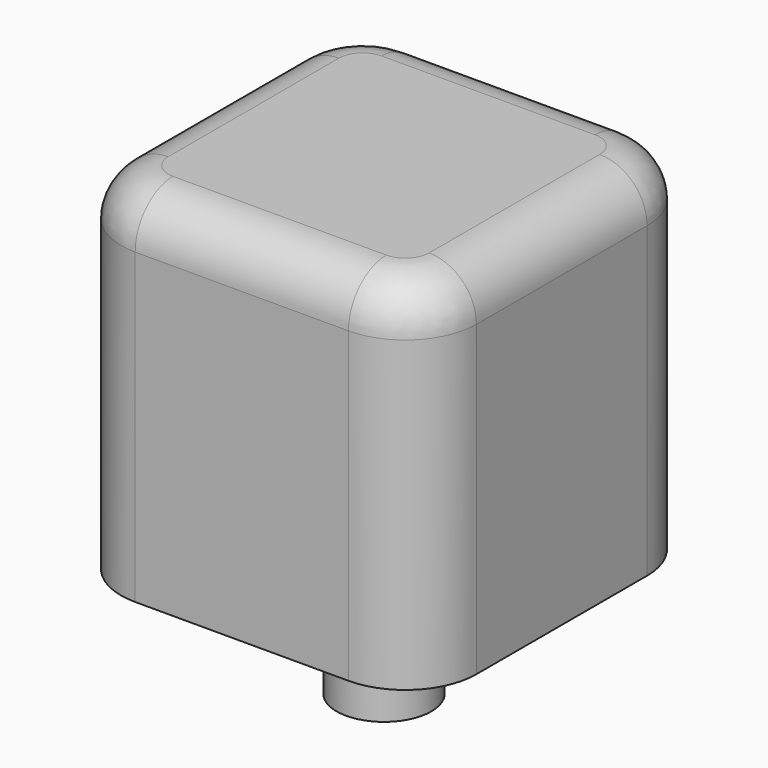
from build123d import *

# Parameters (mm, degrees)
F0_W         = 19.05
F0_H         = 19.05
F1_DEPTH     = 19.05
F2_R         = 2.54
F3_T1_DEPTH  = 28.575
F3_T4_ANGLE  = 90
F3_T6_ANGLE  = 90
F3_T8_ANGLE  = 90
F3_T10_ANGLE = 90
F4_R         = 2.54
F5_DEPTH     = 6.35


# Not quite as in the source:
# - a fillet or chamfer that OpenCascade refuses, or shapes differently, is made with other operations: its cross-section is extruded or revolved along the edge and cut away or added


with BuildPart() as f1:
    # F0 (on Top) → F1 (new body)
    with BuildSketch(Plane.XY):
        with Locations((-40.0474531332, 35.1082887501)):
            Rectangle(F0_W, F0_H)
    extrude(amount=F1_DEPTH)

    # F2
    f2_edges = [f1.edges().sort_by_distance(p)[0] for p in [
        (-40.047453, 44.633289, 19.05),
        (-49.572453, 35.108289, 19.05),
        (-40.047453, 25.583289, 19.05),
        (-30.522453, 35.108289, 19.05),
    ]]
    fillet(f2_edges, radius=F2_R)

    # F3: fillet of radius 3.81 on 4 edges, made by hand

    # F3_s2 → F3_t1 (cut)
    with BuildSketch(Plane.XY.offset(-9.525)):
        with BuildLine():
            ThreePointArc((-49.5724531332, 29.3932887501), (-48.4565299695, 26.6992119137), (-45.7624531332, 25.5832887501))
            Line((-45.7624531332, 25.5832887501), (-49.5724531332, 25.5832887501))
            Line((-49.5724531332, 25.5832887501), (-49.5724531332, 29.3932887501))
        make_face()
        with BuildLine():
            ThreePointArc((-45.7624531332, 44.6332887501), (-48.4565299695, 43.5173655864), (-49.5724531332, 40.8232887501))
            Line((-49.5724531332, 40.8232887501), (-49.5724531332, 44.6332887501))
            Line((-49.5724531332, 44.6332887501), (-45.7624531332, 44.6332887501))
        make_face()
        with BuildLine():
            ThreePointArc((-30.5224531332, 29.3932887501), (-31.6383762969, 26.6992119137), (-34.3324531332, 25.5832887501))
            Line((-34.3324531332, 25.5832887501), (-30.5224531332, 25.5832887501))
            Line((-30.5224531332, 25.5832887501), (-30.5224531332, 29.3932887501))
        make_face()
        with BuildLine():
            ThreePointArc((-34.3324531332, 44.6332887501), (-31.6383762969, 43.5173655864), (-30.5224531332, 40.8232887501))
            Line((-30.5224531332, 40.8232887501), (-30.5224531332, 44.6332887501))
            Line((-30.5224531332, 44.6332887501), (-34.3324531332, 44.6332887501))
        make_face()
    extrude(amount=F3_T1_DEPTH, mode=Mode.SUBTRACT)

    # F3_s3 → F3_t4 (revolve, cut)
    with BuildSketch(Plane.XZ.offset(-40.8232887501)):
        with BuildLine():
            ThreePointArc((-33.0624531332, 19.05), (-31.266401909, 18.3060512242), (-30.5224531332, 16.51))
            Line((-30.5224531332, 16.51), (-30.5224531332, 19.05))
            Line((-30.5224531332, 19.05), (-33.0624531332, 19.05))
        make_face()
    revolve(axis=Axis((-34.3324531332, 40.8232887501, 19.05), (0, 0, 1)), revolution_arc=F3_T4_ANGLE, mode=Mode.SUBTRACT)

    # F3_s5 → F3_t6 (revolve, cut)
    with BuildSketch(Plane.YZ.offset(-34.3324531332)):
        with BuildLine():
            ThreePointArc((28.1232887501, 19.05), (26.3272375258, 18.3060512242), (25.5832887501, 16.51))
            Line((25.5832887501, 16.51), (25.5832887501, 19.05))
            Line((25.5832887501, 19.05), (28.1232887501, 19.05))
        make_face()
    revolve(axis=Axis((-34.3324531332, 29.3932887501, 19.05), (0, 0, 1)), revolution_arc=F3_T6_ANGLE, mode=Mode.SUBTRACT)

    # F3_s7 → F3_t8 (revolve, cut)
    with BuildSketch(Plane.YZ.offset(-45.7624531332)):
        with BuildLine():
            ThreePointArc((42.0932887501, 19.05), (43.8893399743, 18.3060512242), (44.6332887501, 16.51))
            Line((44.6332887501, 16.51), (44.6332887501, 19.05))
            Line((44.6332887501, 19.05), (42.0932887501, 19.05))
        make_face()
    revolve(axis=Axis((-45.7624531332, 40.8232887501, 19.05), (0, 0, 1)), revolution_arc=F3_T8_ANGLE, mode=Mode.SUBTRACT)

    # F3_s9 → F3_t10 (revolve, cut)
    with BuildSketch(Plane.XZ.offset(-29.3932887501)):
        with BuildLine():
            ThreePointArc((-47.0324531332, 19.05), (-48.8285043574, 18.3060512242), (-49.5724531332, 16.51))
            Line((-49.5724531332, 16.51), (-49.5724531332, 19.05))
            Line((-49.5724531332, 19.05), (-47.0324531332, 19.05))
        make_face()
    revolve(axis=Axis((-45.7624531332, 29.3932887501, 19.05), (0, 0, 1)), revolution_arc=F3_T10_ANGLE, mode=Mode.SUBTRACT)

    # F4 (on face) → F5 (join)
    with BuildSketch(Plane(origin=(0, 0, 0), x_dir=(1, 0, 0), z_dir=(0, 0, -1))):
        with Locations((-40.0474531332, -35.1082887501)):
            Circle(F4_R)
    extrude(amount=F5_DEPTH)


solid = f1.part
